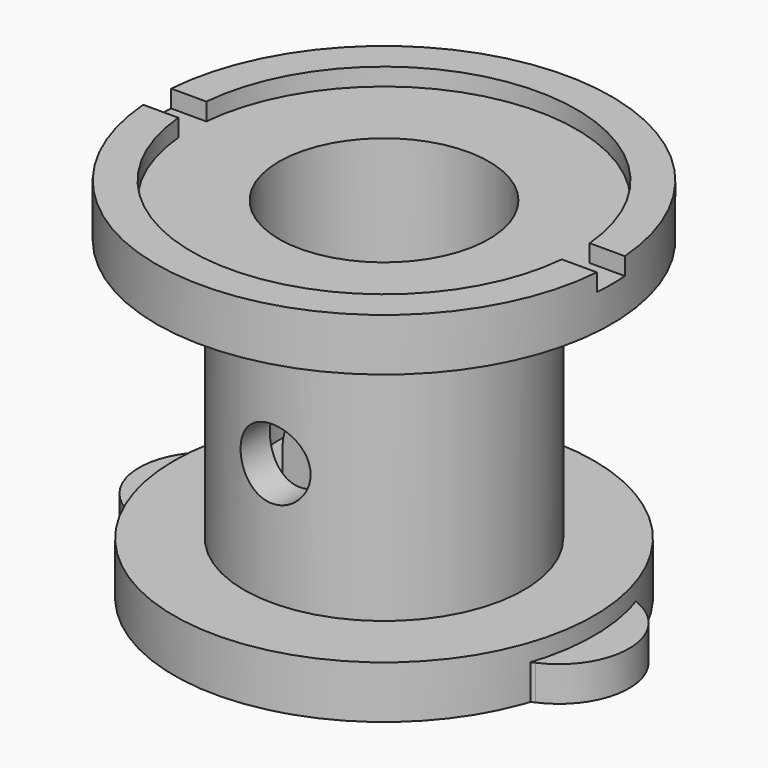
from build123d import *

# Parameters (mm, degrees)
F0_W           = 70
F0_H           = 35
F1_DEPTH       = 10
F3_DEPTH       = 10
F4_R           = 5
F5_R           = 7.5
F6_DEPTH       = 25
F8_DEPTH       = 10.001
F11_R          = 10
F12_DEPTH      = 65.001
F12_DEPTH_BACK = 65.001
F13_W          = 10
F13_H          = 5
F14_DEPTH      = 65.001
F14_DEPTH_BACK = 65.001
F15_R          = 7.5
F16_DEPTH      = 10
F17_R          = 30
F17_R_2        = 20
F18_DEPTH      = 20
F19_DEPTH      = 10.0010001


with BuildPart() as f1:
    # F0 (on Top) → F1 (new body)
    with BuildSketch(Plane.XY):
        Rectangle(F0_W, F0_H)
    extrude(amount=F1_DEPTH)

    # F2 (on face) → F3 (join)
    with BuildSketch(Plane.XZ.offset(17.5)):
        with BuildLine():
            Line((-15, 40), (-15, 10))
            Line((-15, 10), (15, 10))
            Line((15, 10), (15, 40))
            ThreePointArc((15, 40), (0, 55), (-15, 40))
        make_face()
    extrude(amount=-F3_DEPTH)

    # F4
    f4_edges = [f1.edges().sort_by_distance(p)[0] for p in [
        (-35, -17.5, 5),
        (35, -17.5, 5),
        (35, 17.5, 5),
        (-35, 17.5, 5),
    ]]
    fillet(f4_edges, radius=F4_R)

    # F5 (on face) → F6 (cut)
    with BuildSketch(Plane.XZ.offset(17.5)):
        with Locations((0, 40)):
            Circle(F5_R)
    extrude(amount=-F6_DEPTH, mode=Mode.SUBTRACT)

    # F7 (on face) → F8 (cut, through all)
    with BuildSketch(Plane.XY.offset(10)):
        with BuildLine():
            ThreePointArc((21.5, -7.5), (25, -11), (28.5, -7.5))
            Line((28.5, -7.5), (28.5, 7.5))
            ThreePointArc((28.5, 7.5), (25, 11), (21.5, 7.5))
            Line((21.5, 7.5), (21.5, -7.5))
        make_face()
        with BuildLine():
            Line((-28.5, 7.5), (-28.5, -7.5))
            ThreePointArc((-28.5, -7.5), (-25, -11), (-21.5, -7.5))
            Line((-21.5, -7.5), (-21.5, 7.5))
            ThreePointArc((-21.5, 7.5), (-25, 11), (-28.5, 7.5))
        make_face()
    extrude(amount=-F8_DEPTH, mode=Mode.SUBTRACT)


with BuildPart() as f10:
    # F9 (on Front) → F10 (revolve)
    with BuildSketch(Plane.XZ):
        Polygon((-60, 15), (-60, 0), (-30, 0), (-30, 100), (-55, 100), (-55, 105), (-65, 105), (-65, 90), (-40, 90), (-40, 15), align=None)
    revolve(axis=Axis((0, 0, 5.9435109548), (0, 0, -1)))

    # F11 (on Front) → F12 (cut, two sides)
    with BuildSketch(Plane.XZ) as f12_sk:
        with Locations((0, 50)):
            Circle(F11_R)
    extrude(amount=-F12_DEPTH, mode=Mode.SUBTRACT)
    extrude(f12_sk.sketch, amount=F12_DEPTH_BACK, mode=Mode.SUBTRACT)

    # F13 (on Right) → F14 (cut, two sides)
    with BuildSketch(Plane.YZ) as f14_sk:
        with Locations((0, 102.5)):
            Rectangle(F13_W, F13_H)
    extrude(amount=-F14_DEPTH, mode=Mode.SUBTRACT)
    extrude(f14_sk.sketch, amount=F14_DEPTH_BACK, mode=Mode.SUBTRACT)


with BuildPart() as f16:
    # F15 (on Top) → F16 (new body)
    with BuildSketch(Plane.XY):
        with BuildLine():
            ThreePointArc((16, 36.6606055596), (8.1723857476, 39.1562525172), (0, 40))
            ThreePointArc((0, 40), (-8.1723857476, 39.1562525172), (-16, 36.6606055596))
            Line((-16, 36.6606055596), (-58, 18.3303027798))
            ThreePointArc((-58, 18.3303027798), (-70, 0), (-58, -18.3303027798))
            Line((-58, -18.3303027798), (-16, -36.6606055596))
            ThreePointArc((-16, -36.6606055596), (-8.1723857476, -39.1562525172), (0, -40))
            ThreePointArc((0, -40), (8.1723857476, -39.1562525172), (16, -36.6606055596))
            Line((16, -36.6606055596), (58, -18.3303027798))
            ThreePointArc((58, -18.3303027798), (70, 0), (58, 18.3303027798))
            Line((58, 18.3303027798), (16, 36.6606055596))
        make_face()
        with Locations((-50, 0)):
            Circle(F15_R, mode=Mode.SUBTRACT)
        with Locations((50, 0)):
            Circle(F15_R, mode=Mode.SUBTRACT)
    extrude(amount=F16_DEPTH)

    # F17 (on face) → F18 (join)
    with BuildSketch(Plane.XY.offset(10)):
        Circle(F17_R)
        Circle(F17_R_2, mode=Mode.SUBTRACT)
    extrude(amount=F18_DEPTH)

    # F19 (cut, through all): a face of the model
    f19_faces = [f16.faces().sort_by_distance(p)[0] for p in [
        (0, 0, 10),
    ]]
    extrude(f19_faces, amount=-F19_DEPTH, mode=Mode.SUBTRACT)


solid = Compound([f1.part, f10.part, f16.part])
